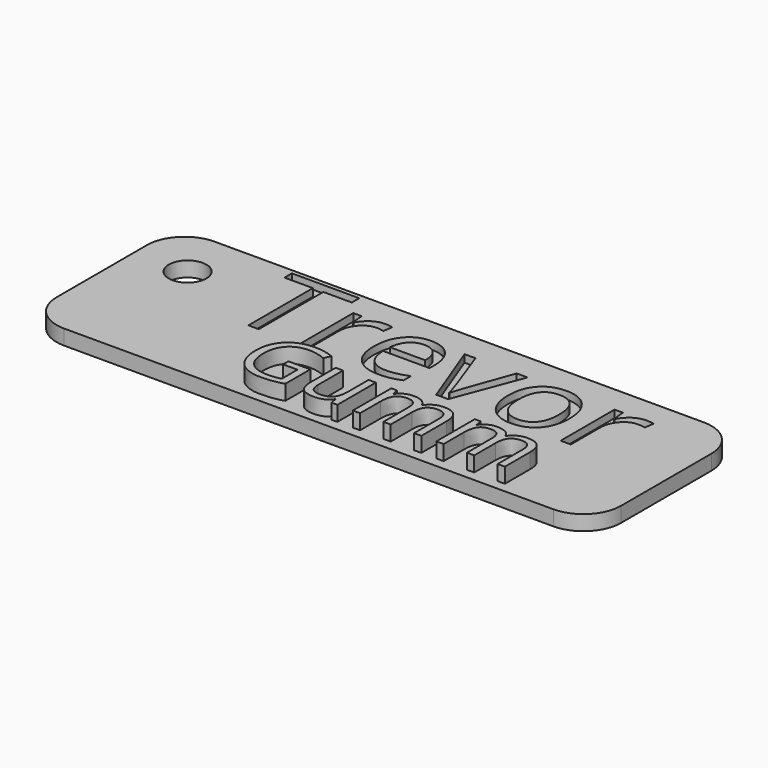
from build123d import *

# Parameters (mm, degrees)
F1_DEPTH     = 2
F3_D         = 5
F4_TEXT_SIZE = 16.7349728549
F5_DEPTH     = 1
F6_TEXT_SIZE = 11.9320902741
F7_DEPTH     = 2


# Not quite as in the source:
# - Text() gives the source's letters only with a copy of the font that has no kerning and outlines rounded to 1/6400 em; it was checked with that copy


with BuildPart() as f1:
    # F0 (on Top) → F1 (new body)
    with BuildSketch(Plane.XY):
        with BuildLine():
            Line((-32.5, -12.5), (32.5, -12.5))
            ThreePointArc((32.5, -12.5), (36.0355339059, -11.0355339059), (37.5, -7.5))
            Line((37.5, -7.5), (37.5, 7.5))
            ThreePointArc((37.5, 7.5), (36.0355339059, 11.0355339059), (32.5, 12.5))
            Line((32.5, 12.5), (-32.5, 12.5))
            ThreePointArc((-32.5, 12.5), (-36.0355339059, 11.0355339059), (-37.5, 7.5))
            Line((-37.5, 7.5), (-37.5, -7.5))
            ThreePointArc((-37.5, -7.5), (-36.0355339059, -11.0355339059), (-32.5, -12.5))
        make_face()
    extrude(amount=F1_DEPTH)

    # F3 (through all)
    with Locations(Plane(origin=(0, 0, 0), x_dir=(1, 0, 0), z_dir=(0, 0, -1))):
        with Locations((-30.5, -5.5)):
            Hole(F3_D / 2)

    # F4 (on face) → F5 (cut)
    with BuildSketch(Plane.XY.offset(2)):
        with Locations((-21.9467226416, 0)):
            Text('Trevor', F4_TEXT_SIZE, font='Open Sans', text_align=(TextAlign.LEFT, TextAlign.BOTTOM))
    extrude(amount=-F5_DEPTH, mode=Mode.SUBTRACT)

    # F6 (on face) → F7 (join)
    with BuildSketch(Plane.XY.offset(2)):
        with Locations((-12.2420173138, -11.1721083522)):
            Text('Gumm', F6_TEXT_SIZE, font='Open Sans', text_align=(TextAlign.LEFT, TextAlign.BOTTOM))
    extrude(amount=F7_DEPTH)


solid = f1.part
